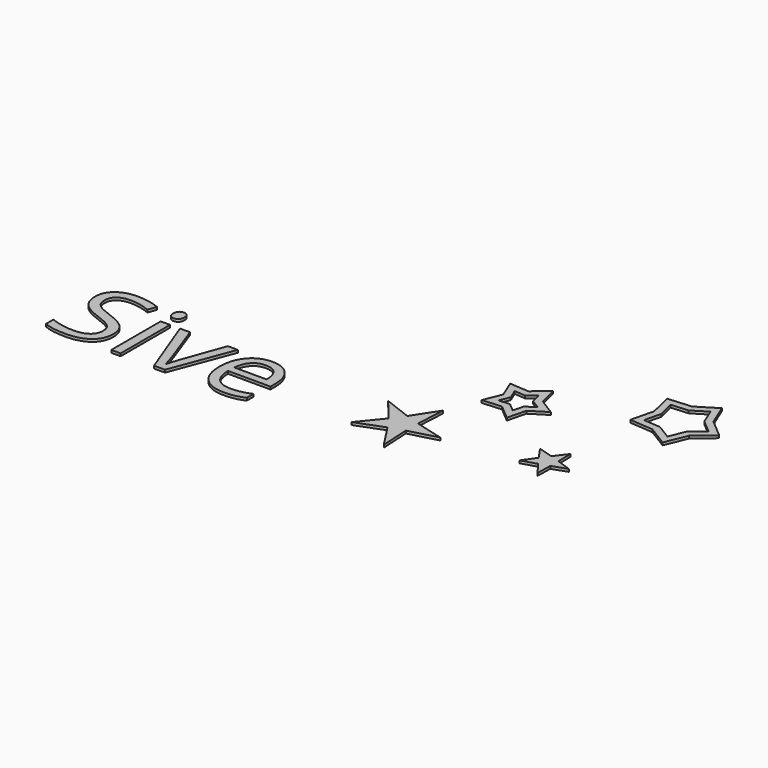
from build123d import *

# Parameters (mm, degrees)
F0_TEXT_SIZE = 13.3233408277
F1_DEPTH     = 0.3


# Not quite as in the source:
# - Text() gives the source's letters only with a copy of the font that has no kerning and outlines rounded to 1/6400 em; it was checked with that copy


with BuildPart() as f1:
    # F0 (on Top) → F1 (new body)
    with BuildSketch(Plane.XY):
        Polygon((45.5197678753, 19.2148680571), (42.8062423837, 19.0067321436), (43.4468188584, 16.3616985083), (42.8062423837, 13.7166648729), (45.5197678753, 13.5085289594), (47.8373953331, 12.0819441849), (48.8738698415, 14.5983427514), (50.9468188584, 16.3616985083), (48.8738698415, 18.1250542651), (47.8373953331, 20.6414528316), align=None)
        Polygon((47.4558552841, 19.467193304), (48.2079466306, 17.641232732), (49.7121293236, 16.3616985083), (48.2079466306, 15.0821642845), (47.4558552841, 13.2562037126), (45.7741279079, 14.2913686445), (43.8051272001, 14.4423971726), (44.2699452149, 16.3616985083), (43.8051272001, 18.2809998439), (45.7741279079, 18.4320283721), align=None, mode=Mode.SUBTRACT)
        Polygon((32.15595247, 12.3196945685), (29.9424269785, 12.4748299189), (30.7739864588, 10.4175815359), (29.9424269785, 8.3603331529), (32.15595247, 8.5154685033), (33.8555459391, 7.0888837288), (34.3920204475, 9.2420110313), (36.2739864588, 10.4175815359), (34.3920204475, 11.5931520405), (33.8555459391, 13.7462793429), align=None)
        Polygon((33.3889164299, 12.3101413844), (33.6939336388, 11.0859622857), (34.7639416466, 10.4175815359), (33.6939336388, 9.7492007861), (33.3889164299, 8.5250216874), (32.4225979039, 9.3361187653), (31.1640788938, 9.2479152238), (31.6368692086, 10.4175815359), (31.1640788938, 11.587247848), (32.4225979039, 11.4990443064), align=None, mode=Mode.SUBTRACT)
        Polygon((41.6785921238, 3.7183704865), (39.9650666323, 4.236777101), (40.9876091182, 2.7673139703), (39.9650666323, 1.2978508395), (41.6785921238, 1.816257454), (42.7601516042, 0.3896726795), (42.7966261126, 2.179528718), (44.4876091182, 2.7673139703), (42.7966261126, 3.3550992225), (42.7601516042, 5.144955261), align=None)
        Polygon((26.6473156337, 1.7384390408), (23.4702646506, 2.9568879016), (25.6108411252, 0.3118542663), (23.4702646506, -2.333179369), (26.6473156337, -1.1147305081), (28.5014175999, -3.967900057), (28.3243666168, -0.5698236121), (31.6108411252, 0.3118542663), (28.3243666168, 1.1935321448), (28.5014175999, 4.5916085897), align=None)
        with Locations((-10.7009347994, -4.8537606961)):
            Text('Sive', F0_TEXT_SIZE, font='Open Sans', text_align=(TextAlign.LEFT, TextAlign.BOTTOM))
    extrude(amount=F1_DEPTH)


solid = f1.part
